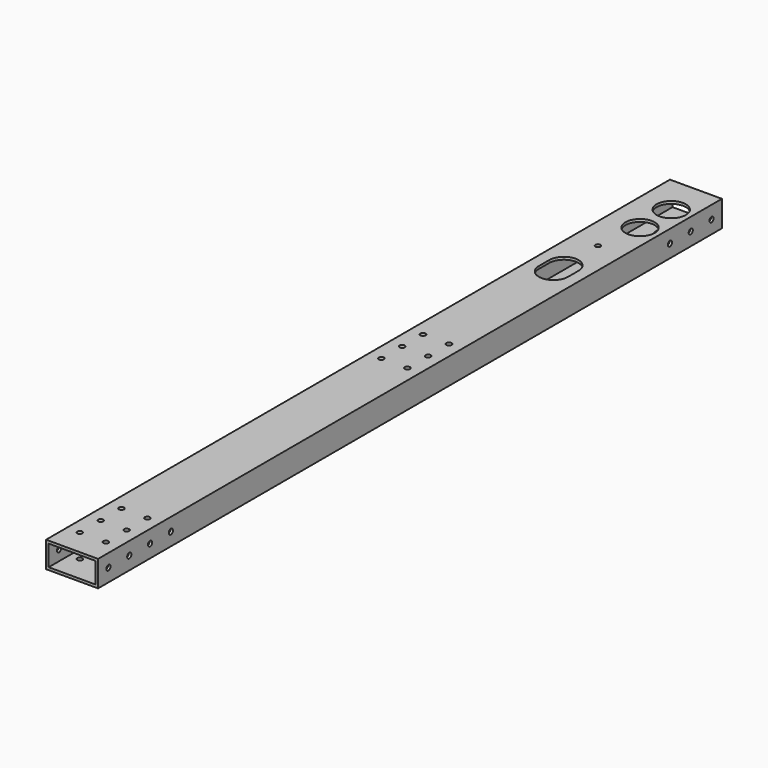
from build123d import *

# Parameters (mm, degrees)
F0_W     = 50.8
F0_H     = 25.4
F0_W_2   = 45.72
F0_H_2   = 20.32
F1_DEPTH = 787.4
F3_R     = 14.2875
F3_R_2   = 2.4892
F3_R_3   = 2.5527
F4_DEPTH = 25.4
F2_R     = 2.5527
F5_DEPTH = 50.801
F6_DEPTH = 25.4


# Not quite as in the source:
# - a feature names something its author has since deleted; it is built from what else it names


with BuildPart() as f1:
    # F0 (on Front) → F1 (new body)
    with BuildSketch(Plane.XZ):
        with Locations((25.4, 12.7)):
            Rectangle(F0_W, F0_H)
        with Locations((25.4, 12.7)):
            Rectangle(F0_W_2, F0_H_2, mode=Mode.SUBTRACT)
    extrude(amount=F1_DEPTH)

    # F3 (on face) → F4 (cut)
    with BuildSketch(Plane.XY.offset(25.4)):
        with Locations((31.75, -63.5)):
            Circle(F3_R)
        with BuildLine():
            ThreePointArc((38.1988341754, -193.04), (39.3103558461, -189.9510821033), (39.6875, -186.69))
            ThreePointArc((39.6875, -186.69), (25.4, -172.4025), (11.1125, -186.69))
            ThreePointArc((11.1125, -186.69), (11.4896441539, -189.9510821033), (12.6011658246, -193.04))
            ThreePointArc((12.6011658246, -193.04), (25.4, -185.1025), (38.1988341754, -193.04))
        make_face()
        with BuildLine():
            Line((39.6875, -199.39), (39.6875, -186.69))
            ThreePointArc((39.6875, -186.69), (39.3103558461, -189.9510821033), (38.1988341754, -193.04))
            ThreePointArc((38.1988341754, -193.04), (39.3103558461, -196.1289178967), (39.6875, -199.39))
        make_face()
        with BuildLine():
            ThreePointArc((12.6011658246, -193.04), (11.4896441539, -189.9510821033), (11.1125, -186.69))
            Line((11.1125, -186.69), (11.1125, -199.39))
            ThreePointArc((11.1125, -199.39), (11.4896441539, -196.1289178967), (12.6011658246, -193.04))
        make_face()
        with BuildLine():
            ThreePointArc((39.6875, -199.39), (39.3103558461, -196.1289178967), (38.1988341754, -193.04))
            ThreePointArc((38.1988341754, -193.04), (25.4, -200.9775), (12.6011658246, -193.04))
            ThreePointArc((12.6011658246, -193.04), (11.4896441539, -196.1289178967), (11.1125, -199.39))
            ThreePointArc((11.1125, -199.39), (25.4, -213.6775), (39.6875, -199.39))
        make_face()
        with BuildLine():
            ThreePointArc((12.6011658246, -193.04), (25.4, -200.9775), (38.1988341754, -193.04))
            ThreePointArc((38.1988341754, -193.04), (25.4, -185.1025), (12.6011658246, -193.04))
        make_face()
        with Locations((12.7, -736.6)):
            Circle(F3_R_2)
        with Locations((12.7, -711.2)):
            Circle(F3_R_2)
        with Locations((38.1, -736.6)):
            Circle(F3_R_2)
        with Locations((38.1, -711.2)):
            Circle(F3_R_2)
        with Locations((12.7, -342.9)):
            Circle(F3_R_3)
        with Locations((12.7, -368.3)):
            Circle(F3_R_3)
        with Locations((12.7, -393.7)):
            Circle(F3_R_3)
        with Locations((38.1, -342.9)):
            Circle(F3_R_3)
        with Locations((38.1, -368.3)):
            Circle(F3_R_3)
        with Locations((38.1, -393.7)):
            Circle(F3_R_3)
        with Locations((25.4, -145.034)):
            Circle(F3_R_2)
        with Locations((38.1, -762)):
            Circle(F3_R_2)
        with Locations((12.7, -762)):
            Circle(F3_R_2)
        with Locations((31.75, -101.6)):
            Circle(F3_R)
    extrude(amount=-F4_DEPTH, mode=Mode.SUBTRACT)

    # F2 (on face) → F5 (cut, through all)
    with BuildSketch(Plane.YZ.offset(50.8)):
        with Locations((-12.7, 12.7)):
            Circle(F2_R)
        with Locations((-38.1, 12.7)):
            Circle(F2_R)
        with Locations((-63.5, 12.7)):
            Circle(F2_R)
        with Locations((-88.9, 12.7)):
            Circle(F2_R)
        with Locations((-774.7, 12.7)):
            Circle(F2_R)
        with Locations((-749.3, 12.7)):
            Circle(F2_R)
        with Locations((-723.9, 12.7)):
            Circle(F2_R)
        with Locations((-698.5, 12.7)):
            Circle(F2_R)
    extrude(amount=-F5_DEPTH, mode=Mode.SUBTRACT)

    # F0 (on Front) → F6 (cut)
    with BuildSketch(Plane.XZ):
        with Locations((25.4, 12.7)):
            Rectangle(F0_W, F0_H)
        with Locations((25.4, 12.7)):
            Rectangle(F0_W_2, F0_H_2, mode=Mode.SUBTRACT)
    extrude(amount=F6_DEPTH, mode=Mode.SUBTRACT)


solid = f1.part
